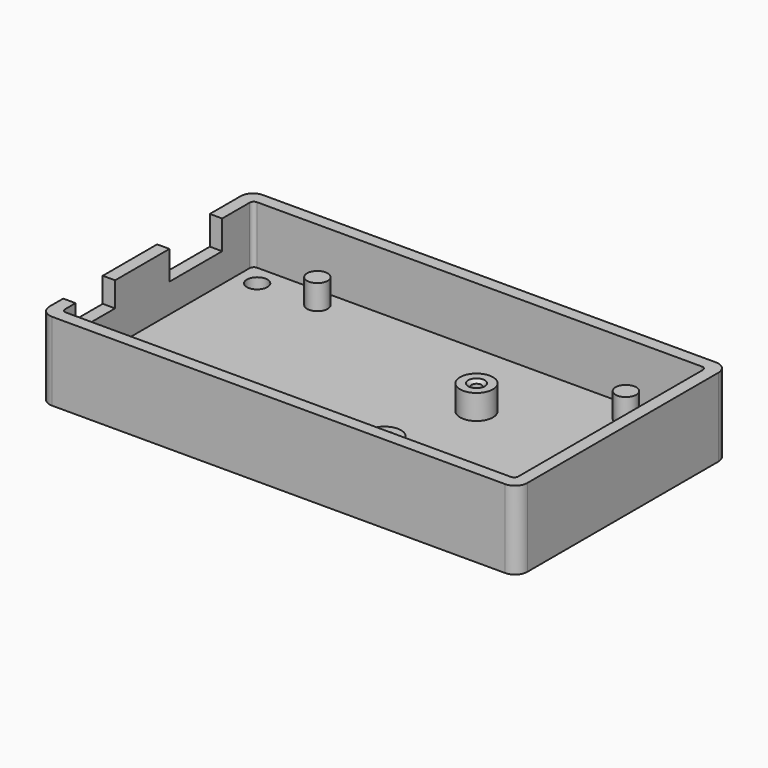
from build123d import *

# Parameters (mm, degrees)
F2_DEPTH       = 5
F4_DEPTH       = 14
F3_R           = 2.5
F3_R_2         = 4
F5_DEPTH       = 6
F7_D           = 2.5
F7_DEPTH       = 6
F7_CSINK_D     = 4
F7_CSINK_ANGLE = 90
F7_TIP         = 0.7510757738
F8_D           = 5
F9_W           = 16
F9_H           = 7
F9_W_2         = 12
F9_H_2         = 6
F10_DEPTH      = 3


# Not quite as in the source:
# - a feature names something its author has since deleted; it is built from what else it names


with BuildPart() as f2:
    # F1 (on Top) → F2 (new body)
    with BuildSketch(Plane.XY):
        with BuildLine():
            ThreePointArc((58, 29), (57.1213203436, 31.1213203436), (55, 32))
            Line((55, 32), (-55, 32))
            ThreePointArc((-55, 32), (-57.1213203436, 31.1213203436), (-58, 29))
            Line((-58, 29), (-58, -29))
            ThreePointArc((-58, -29), (-57.1213203436, -31.1213203436), (-55, -32))
            Line((-55, -32), (55, -32))
            ThreePointArc((55, -32), (57.1213203436, -31.1213203436), (58, -29))
            Line((58, -29), (58, 29))
        make_face()
        with BuildLine():
            ThreePointArc((55, -28), (54.7071067812, -28.7071067812), (54, -29))
            Line((54, -29), (-54, -29))
            ThreePointArc((-54, -29), (-54.7071067812, -28.7071067812), (-55, -28))
            Line((-55, -28), (-55, 28))
            ThreePointArc((-55, 28), (-54.7071067812, 28.7071067812), (-54, 29))
            Line((-54, 29), (54, 29))
            ThreePointArc((54, 29), (54.7071067812, 28.7071067812), (55, 28))
            Line((55, 28), (55, -28))
        make_face(mode=Mode.SUBTRACT)
        with BuildLine():
            Line((-54, -29), (54, -29))
            ThreePointArc((54, -29), (54.7071067812, -28.7071067812), (55, -28))
            Line((55, -28), (55, 28))
            ThreePointArc((55, 28), (54.7071067812, 28.7071067812), (54, 29))
            Line((54, 29), (-54, 29))
            ThreePointArc((-54, 29), (-54.7071067812, 28.7071067812), (-55, 28))
            Line((-55, 28), (-55, -28))
            ThreePointArc((-55, -28), (-54.7071067812, -28.7071067812), (-54, -29))
        make_face()
    extrude(amount=F2_DEPTH)

    # F3 (on face) → F4 (join)
    with BuildSketch(Plane.XY.offset(5)):
        with BuildLine():
            ThreePointArc((58, 29), (57.1213203436, 31.1213203436), (55, 32))
            Line((55, 32), (-55, 32))
            ThreePointArc((-55, 32), (-57.1213203436, 31.1213203436), (-58, 29))
            Line((-58, 29), (-58, -29))
            ThreePointArc((-58, -29), (-57.1213203436, -31.1213203436), (-55, -32))
            Line((-55, -32), (55, -32))
            ThreePointArc((55, -32), (57.1213203436, -31.1213203436), (58, -29))
            Line((58, -29), (58, 29))
        make_face()
        with BuildLine():
            ThreePointArc((55, -28), (54.7071067812, -28.7071067812), (54, -29))
            Line((54, -29), (-54, -29))
            ThreePointArc((-54, -29), (-54.7071067812, -28.7071067812), (-55, -28))
            Line((-55, -28), (-55, 28))
            ThreePointArc((-55, 28), (-54.7071067812, 28.7071067812), (-54, 29))
            Line((-54, 29), (54, 29))
            ThreePointArc((54, 29), (54.7071067812, 28.7071067812), (55, 28))
            Line((55, 28), (55, -28))
        make_face(mode=Mode.SUBTRACT)
    extrude(amount=F4_DEPTH)

    # F3 (on face) → F5 (join)
    with BuildSketch(Plane.XY.offset(5)):
        with BuildLine():
            ThreePointArc((58, 29), (57.1213203436, 31.1213203436), (55, 32))
            Line((55, 32), (-55, 32))
            ThreePointArc((-55, 32), (-57.1213203436, 31.1213203436), (-58, 29))
            Line((-58, 29), (-58, -29))
            ThreePointArc((-58, -29), (-57.1213203436, -31.1213203436), (-55, -32))
            Line((-55, -32), (55, -32))
            ThreePointArc((55, -32), (57.1213203436, -31.1213203436), (58, -29))
            Line((58, -29), (58, 29))
        make_face()
        with BuildLine():
            ThreePointArc((55, -28), (54.7071067812, -28.7071067812), (54, -29))
            Line((54, -29), (-54, -29))
            ThreePointArc((-54, -29), (-54.7071067812, -28.7071067812), (-55, -28))
            Line((-55, -28), (-55, 28))
            ThreePointArc((-55, 28), (-54.7071067812, 28.7071067812), (-54, 29))
            Line((-54, 29), (54, 29))
            ThreePointArc((54, 29), (54.7071067812, 28.7071067812), (55, 28))
            Line((55, 28), (55, -28))
        make_face(mode=Mode.SUBTRACT)
        with Locations((-35.5, 24.15)):
            Circle(F3_R)
        with Locations((-36.8, -24.15)):
            Circle(F3_R)
        with Locations((15.3, 8.95)):
            Circle(F3_R_2)
        with Locations((15.3, -18.95)):
            Circle(F3_R_2)
        with Locations((45.95, -24.15)):
            Circle(F3_R)
        with Locations((39.4, 24.15)):
            Circle(F3_R)
    extrude(amount=F5_DEPTH)

    # F7
    with Locations(Plane.XY.offset(11)):
        with Locations((15.3, 8.95), (15.3, -18.95)):
            CounterSinkHole(F7_D / 2, F7_CSINK_D / 2, depth=F7_DEPTH, counter_sink_angle=F7_CSINK_ANGLE)
            with Locations((0, 0, -(F7_DEPTH + F7_TIP / 2))):  # 118° drill point
                Cone(0, F7_D / 2, F7_TIP, mode=Mode.SUBTRACT)

    # F8 (through all)
    with Locations(Plane.XY.offset(5)):
        with Locations((-50, 24), (50, 24), (35.95, -24), (-50, -24)):
            Hole(F8_D / 2)

    # F9 (on face) → F10 (cut, through all)
    with BuildSketch(Plane(origin=(-58, 0, 0), x_dir=(0, -1, 0), z_dir=(-1, 0, 0))):
        with Locations((-11.65, 15.5)):
            Rectangle(F9_W, F9_H)
        with Locations((18.85, 16)):
            Rectangle(F9_W_2, F9_H_2)
    extrude(amount=-F10_DEPTH, mode=Mode.SUBTRACT)


solid = f2.part
